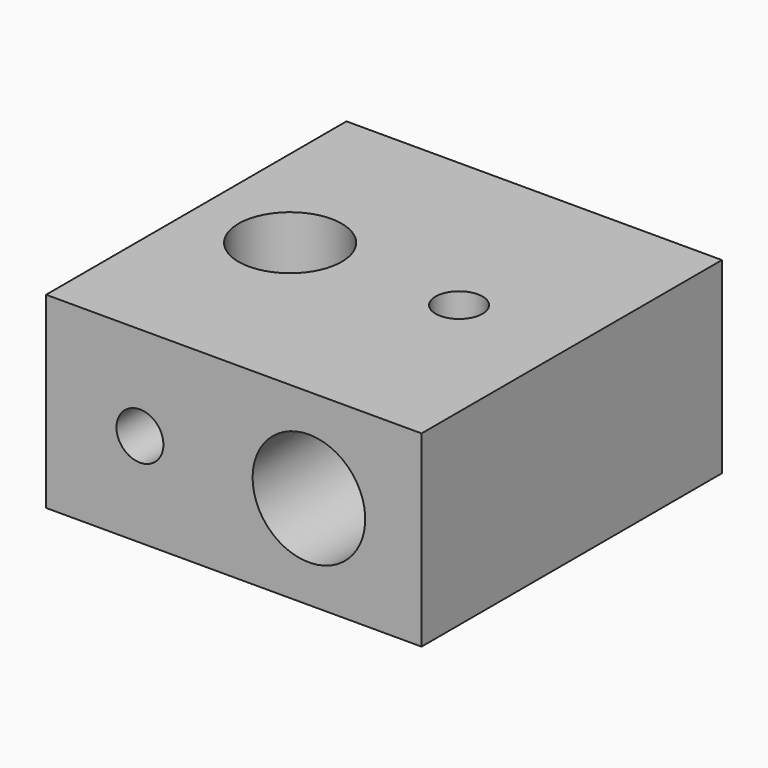
from build123d import *

# Parameters (mm, degrees)
F0_W         = 20
F0_H         = 20
F1_DEPTH     = 10
F3_D         = 6
F4_D         = 2.5
F4_DEPTH     = 6
F4_TIP       = 0.7510757738
F6_D         = 5.5
F7_D         = 2.5
F7_DEPTH     = 3
F7_TIP       = 0.7510757738
F8_TEXT_SIZE = 4.1666666667
F9_DEPTH     = 0.5


# Not quite as in the source:
# - Text() gives the source's letters only with a copy of the font that has no kerning and outlines rounded to 1/6400 em; it was checked with that copy


with BuildPart() as f1:
    # F0 (on Top) → F1 (new body)
    with BuildSketch(Plane.XY):
        with Locations((10, 10)):
            Rectangle(F0_W, F0_H)
    extrude(amount=F1_DEPTH)

    # F3 (through all)
    with Locations(Plane.XZ):
        with Locations((14, 5)):
            Hole(F3_D / 2)

    # F4
    with Locations(Plane.XZ):
        with Locations((5, 5)):
            Hole(F4_D / 2, depth=F4_DEPTH)
            with Locations((0, 0, -(F4_DEPTH + F4_TIP / 2))):  # 118° drill point
                Cone(0, F4_D / 2, F4_TIP, mode=Mode.SUBTRACT)

    # F6 (through all)
    with Locations(Plane.XY.offset(10)):
        with Locations((5, 10)):
            Hole(F6_D / 2)

    # F7
    with Locations(Plane.XY.offset(10)):
        with Locations((14, 10)):
            Hole(F7_D / 2, depth=F7_DEPTH)
            with Locations((0, 0, -(F7_DEPTH + F7_TIP / 2))):  # 118° drill point
                Cone(0, F7_D / 2, F7_TIP, mode=Mode.SUBTRACT)

    # F8 (on face) → F9 (cut)
    with BuildSketch(Plane(origin=(0, 0, 0), x_dir=(1, 0, 0), z_dir=(0, 0, -1))):
        with Locations((9.4016927083, -6.2641595091)):
            Text('UP', F8_TEXT_SIZE, font='Open Sans', text_align=(TextAlign.LEFT, TextAlign.BOTTOM))
    extrude(amount=-F9_DEPTH, mode=Mode.SUBTRACT)


solid = f1.part
